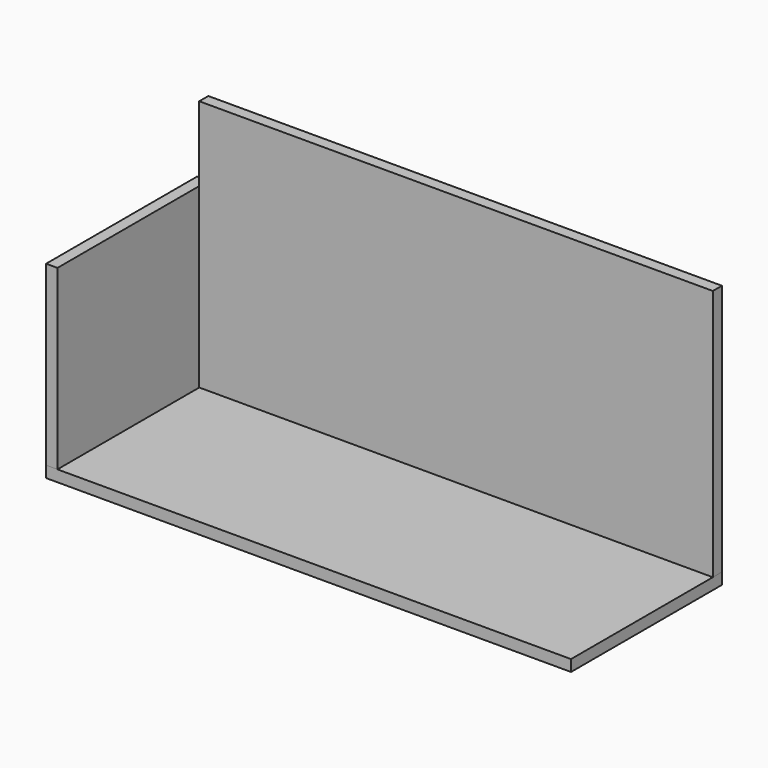
from build123d import *

# Parameters (mm, degrees)
F0_W     = 4520
F0_H     = 1560
F1_DEPTH = 100
F0_H_2   = 100
F2_DEPTH = 2218
F3_DEPTH = 100
F4_DEPTH = 1561
F5_DEPTH = 100


with BuildPart() as f1:
    # F0 (on Top) → F1 (new body)
    with BuildSketch(Plane.XY):
        with Locations((-2260, 780)):
            Rectangle(F0_W, F0_H)
    extrude(amount=-F1_DEPTH)

    # F0 (on Top) → F3 (join)
    with BuildSketch(Plane.XY):
        with Locations((-2260, 1610)):
            Rectangle(F0_W, F0_H_2)
    extrude(amount=-F3_DEPTH)

    # F0 (on Top) → F5 (join)
    with BuildSketch(Plane.XY):
        Polygon((-4620, 0), (-4520, 0), (-4520, 1560), (-4520, 1660), (-4620, 1660), align=None)
    extrude(amount=-F5_DEPTH)


with BuildPart() as f2:
    # F0 (on Top) → F2 (new body)
    with BuildSketch(Plane.XY):
        with Locations((-2260, 1610)):
            Rectangle(F0_W, F0_H_2)
    extrude(amount=F2_DEPTH)


with BuildPart() as f4:
    # F0 (on Top) → F4 (new body)
    with BuildSketch(Plane.XY):
        Polygon((-4620, 0), (-4520, 0), (-4520, 1560), (-4520, 1660), (-4620, 1660), align=None)
    extrude(amount=F4_DEPTH)


solid = Compound([f1.part, f2.part, f4.part])
